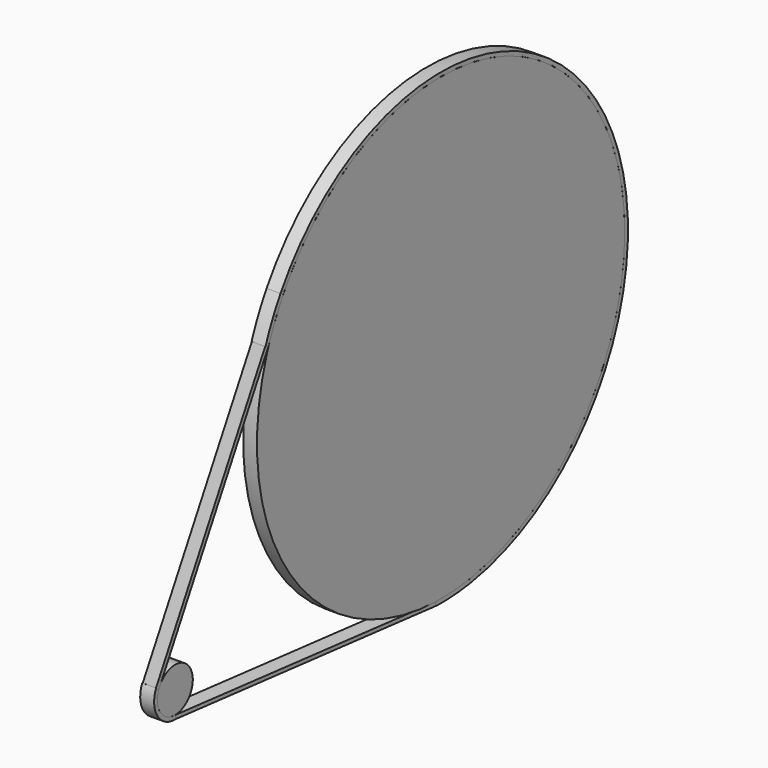
from build123d import *

# Parameters (mm, degrees)
F0_R      = 285.3309
F1_DEPTH  = 8.636
F4_R      = 27.4999958
F5_DEPTH  = 17.272
F9_DEPTH  = 17.272
F12_DEPTH = 17.272
F14_DEPTH = 17.272


with BuildPart() as f1:
    # F0 (on Right) → F1 (new body, symmetric)
    with BuildSketch(Plane.YZ):
        Circle(F0_R)
    extrude(amount=F1_DEPTH, both=True)


with BuildPart() as f5:
    # F4 (on plane+point) → F5 (new body)
    with BuildSketch(Plane(origin=(-27.8706326, 0, 0), x_dir=(0, -1, 0), z_dir=(-1, 0, 0))):
        with Locations((366.811433, -247.5421262)):
            Circle(F4_R)
    extrude(amount=F5_DEPTH)


with BuildPart() as f9:
    # F6 (on face) → F9 (new body, through all)
    with BuildSketch(Plane.YZ.offset(8.636)):
        with BuildLine():
            ThreePointArc((45.5478122499, -286.7358162038), (240.6572930034, 162.4072006381), (-248.8641948571, 149.5280709864))
            Line((-248.8641948571, 149.5280709864), (-267.5215065798, 99.2268411875))
            ThreePointArc((-267.5215065798, 99.2268411875), (50.4062012704, 280.8432612122), (285.3309, 0))
            ThreePointArc((285.3309, 0), (198.8819923056, -204.5963724785), (-8.0805435652, -285.2164569419))
            Line((-8.0805435652, -285.2164569419), (45.5478122499, -286.7358162038))
        make_face()
        with BuildLine():
            Line((-267.5215065798, 99.2268411875), (-248.8641948571, 149.5280709864))
            ThreePointArc((-248.8641948571, 149.5280709864), (-261.6658293387, 125.7896070879), (-272.2094234262, 100.965644121))
            Line((-272.2094234262, 100.965644121), (-267.5215065798, 99.2268411875))
        make_face()
        with BuildLine():
            ThreePointArc((-8.2221430829, -290.2144514974), (18.7437088264, -289.725223055), (45.5478122499, -286.7358162038))
            Line((45.5478122499, -286.7358162038), (-8.0805435652, -285.2164569419))
            Line((-8.0805435652, -285.2164569419), (-8.2221430829, -290.2144514974))
        make_face()
    extrude(amount=-F9_DEPTH)

    # F11 (on 3pt) → F12 (join)
    with BuildSketch(Plane(origin=(28.9472699963, -2.9967644368, -2.0223618286), x_dir=(-0.1024770702, -0.9947096022, 0.0071594218), z_dir=(-0.9922908993, 0.1027268574, 0.0693250603))):
        Polygon((366.6379115019, -281.3036351275), (366.5325688778, -276.3047449575), (5.1108173853, -283.921058662), (5.2158850342, -288.9069002593), align=None)
        Polygon((270.6071909513, 101.3220147825), (265.9316262262, 99.5874398647), (391.6702989577, -239.3424597695), (396.3581002221, -237.6033452516), align=None)
    extrude(amount=F12_DEPTH)

    # F13 (on face) → F14 (join)
    with BuildSketch(Plane.YZ.offset(-27.8706326)):
        with BuildLine():
            ThreePointArc((-392.5949717172, -237.9787115264), (-392.2909462423, -237.1959107597), (-391.9631609319, -236.4227579158))
            Line((-391.9631609319, -236.4227579158), (-396.2135714078, -233.6942388503))
            ThreePointArc((-396.2135714078, -233.6942388503), (-393.0036726401, -266.7831321413), (-362.388232945, -279.7397197168))
            Line((-362.388232945, -279.7397197168), (-363.0687253491, -274.786243151))
            ThreePointArc((-363.0687253491, -274.786243151), (-365.3244296393, -275.0018893091), (-367.5902302284, -275.0310920568))
            ThreePointArc((-367.5902302284, -275.0310920568), (-389.6063699042, -262.9252539878), (-392.5949717172, -237.9787115264))
        make_face()
    extrude(amount=-F14_DEPTH)


solid = Compound([f1.part, f5.part, f9.part])
